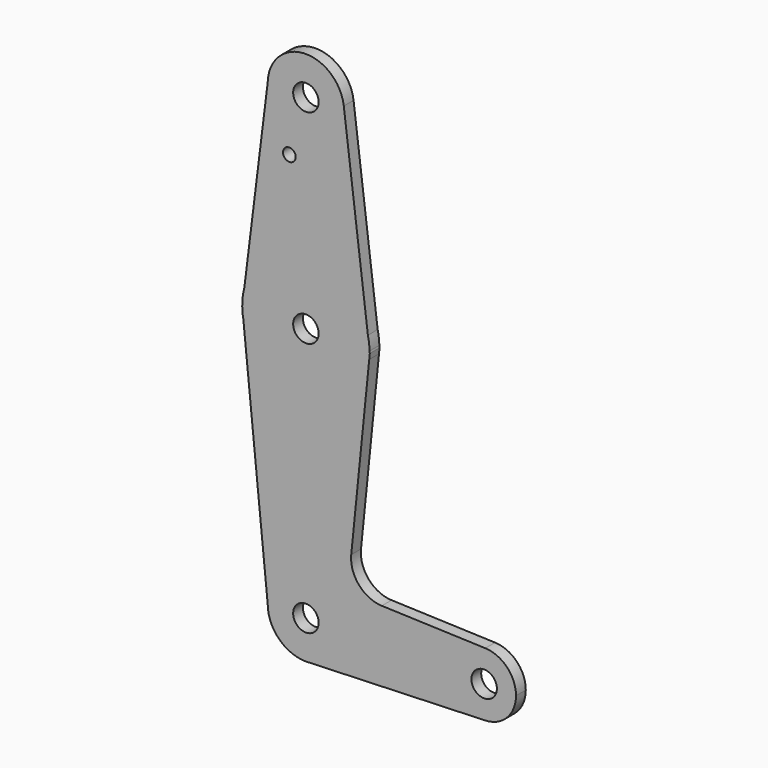
from build123d import *

# Parameters (mm, degrees)
F0_R     = 3.175
F0_R_2   = 1.5875
F1_DEPTH = 3.048


with BuildPart() as f1:
    # F0 (on Front) → F1 (new body)
    with BuildSketch(Plane.XZ):
        with BuildLine():
            ThreePointArc((0.6773435479, -9.500885786), (6.9705567315, -6.4912990883), (9.525, 0))
            ThreePointArc((9.525, 0), (0, 9.525), (-9.525, 0))
            ThreePointArc((-9.525, 0), (-6.7351920908, -6.7351920908), (0, -9.525))
            Line((0, -9.525), (0.6773435479, -9.500885786))
        make_face()
        Circle(F0_R, mode=Mode.SUBTRACT)
        with BuildLine():
            ThreePointArc((-9.525, 0), (0, 9.525), (9.525, 0))
            ThreePointArc((9.525, 0), (6.9705567315, -6.4912990883), (0.6773435479, -9.500885786))
            Line((0.6773435479, -9.500885786), (44.7324052746, -7.9324746146))
            ThreePointArc((44.7324052746, -7.9324746146), (36.5125, 0), (44.7324052746, 7.9324746146))
            Line((44.7324052746, 7.9324746146), (18.9341027877, 8.850924033))
            ThreePointArc((18.9341027877, 8.850924033), (13.2249738114, 11.5709798305), (11.3072231466, 17.5971800924))
            Line((11.3072231466, 17.5971800924), (15.7942028382, 61.9003807621))
            ThreePointArc((15.7942028382, 61.9003807621), (0.6754711443, 47.6393769437), (-15.6010113814, 60.5633234978))
            Line((-15.6010113814, 60.5633234978), (-9.525, 0))
        make_face()
        with BuildLine():
            ThreePointArc((0, -9.525), (0.3388863295, -9.5189695375), (0.6773435479, -9.500885786))
            Line((0.6773435479, -9.500885786), (0, -9.525))
        make_face()
        with BuildLine():
            Line((-15.8734616555, 63.2790020988), (-15.6010113814, 60.5633234978))
            ThreePointArc((-15.6010113814, 60.5633234978), (0.6754711443, 47.6393769437), (15.7942028382, 61.9003807621))
            ThreePointArc((15.7942028382, 61.9003807621), (15.8547878424, 62.6991707598), (15.875, 63.5))
            ThreePointArc((15.875, 63.5), (15.874419829, 63.6357206458), (15.8726793583, 63.7714313715))
            Line((15.8726793583, 63.7714313715), (15.4569841354, 67.1190145672))
            ThreePointArc((15.4569841354, 67.1190145672), (0.2433839863, 79.373134197), (-15.3387626985, 67.5912081197))
            Line((-15.3387626985, 67.5912081197), (-15.8734616555, 63.2790020988))
        make_face()
        with Locations((0, 63.5)):
            Circle(F0_R, mode=Mode.SUBTRACT)
        with BuildLine():
            ThreePointArc((-15.8734616555, 63.2790020988), (-15.795706404, 61.9152968109), (-15.6010113814, 60.5633234978))
            Line((-15.6010113814, 60.5633234978), (-15.8734616555, 63.2790020988))
        make_face()
        with BuildLine():
            ThreePointArc((44.7324052746, 7.9324746146), (36.5125, 0), (44.7324052746, -7.9324746146))
            ThreePointArc((44.7324052746, -7.9324746146), (50.1616327839, -5.5119104847), (52.3875, 0))
            ThreePointArc((52.3875, 0), (50.1616327839, 5.5119104847), (44.7324052746, 7.9324746146))
        make_face()
        with Locations((44.45, 0)):
            Circle(F0_R, mode=Mode.SUBTRACT)
        with BuildLine():
            ThreePointArc((-15.3387626985, 67.5912081197), (-15.7543491606, 65.4534859937), (-15.8734616555, 63.2790020988))
            Line((-15.8734616555, 63.2790020988), (-15.3387626985, 67.5912081197))
        make_face()
        with BuildLine():
            ThreePointArc((15.875, 63.5), (15.8547878424, 62.6991707598), (15.7942028382, 61.9003807621))
            Line((15.7942028382, 61.9003807621), (15.9338280988, 63.2790020988))
            Line((15.9338280988, 63.2790020988), (15.8726793583, 63.7714313715))
            ThreePointArc((15.8726793583, 63.7714313715), (15.874419829, 63.6357206458), (15.875, 63.5))
        make_face()
        with BuildLine():
            Line((-9.5230337628, 114.4935276514), (-15.3387626985, 67.5912081197))
            ThreePointArc((-15.3387626985, 67.5912081197), (0.2433839863, 79.373134197), (15.4569841354, 67.1190145672))
            Line((15.4569841354, 67.1190145672), (9.4524003041, 115.4737774452))
            ThreePointArc((9.4524003041, 115.4737774452), (9.5068327506, 114.8880102479), (9.525, 114.3))
            ThreePointArc((9.525, 114.3), (-0.0967688198, 104.775491572), (-9.5230337628, 114.4935276514))
        make_face()
        with Locations((-4.1181622073, 100.3728732467)):
            Circle(F0_R_2, mode=Mode.SUBTRACT)
        with BuildLine():
            ThreePointArc((15.8726793583, 63.7714313715), (15.7540005069, 65.456295742), (15.4569841354, 67.1190145672))
            Line((15.4569841354, 67.1190145672), (15.8726793583, 63.7714313715))
        make_face()
        with BuildLine():
            ThreePointArc((9.4524003041, 115.4737774452), (-0.4913956511, 123.8123159806), (-9.5230337628, 114.4935276514))
            ThreePointArc((-9.5230337628, 114.4935276514), (-0.0967688198, 104.775491572), (9.525, 114.3))
            ThreePointArc((9.525, 114.3), (9.5068327506, 114.8880102479), (9.4524003041, 115.4737774452))
        make_face()
        with Locations((0, 114.3)):
            Circle(F0_R, mode=Mode.SUBTRACT)
    extrude(amount=F1_DEPTH)


solid = f1.part
